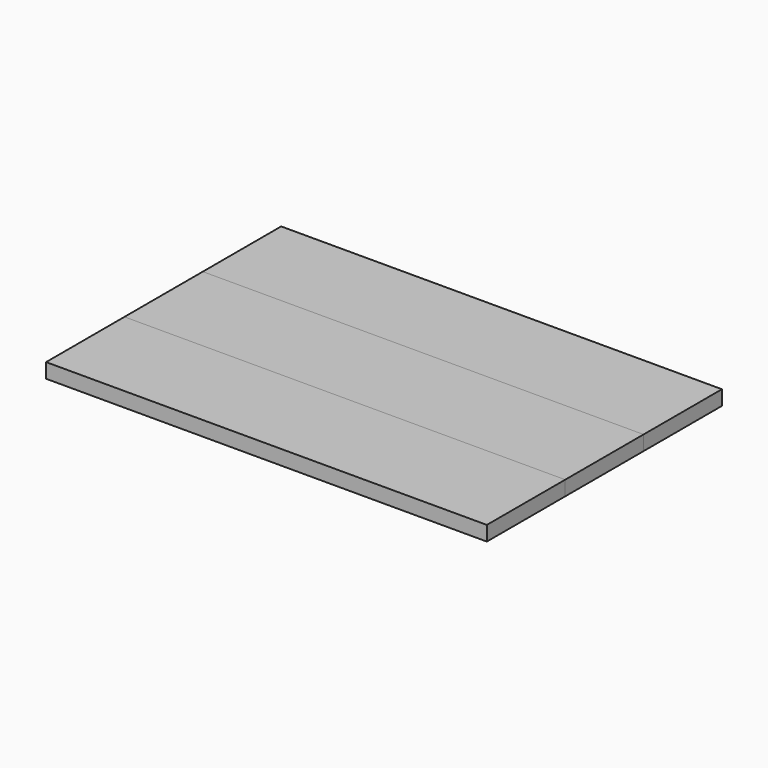
from build123d import *

# Parameters (mm, degrees)
F1_W        = 114.3
F1_H        = 25.4
F3_DEPTH    = 3.81
F4_DEPTH    = 2.54
F5_T1_DEPTH = 13.0403255158


# Not quite as in the source:
# - a fillet or chamfer that OpenCascade refuses, or shapes differently, is made with other operations: its cross-section is extruded or revolved along the edge and cut away or added


with BuildPart() as f3:
    # F1 (on Top) → F3 (new body)
    with BuildSketch(Plane.XY):
        Rectangle(F1_W, F1_H)
    extrude(amount=F3_DEPTH)

    # F2 (on face) → F4 (cut)
    with BuildSketch(Plane.XY):
        Polygon((15.875, 4.7625), (15.875, 3.175), (-15.875, 3.175), (-15.875, 4.7625), (-50.8, 4.7625), (-50.8, -4.7625), (-15.875, -4.7625), (-15.875, -3.175), (15.875, -3.175), (15.875, -4.7625), (50.8, -4.7625), (50.8, 4.7625), align=None)
    extrude(amount=F4_DEPTH, mode=Mode.SUBTRACT)

    # F5: fillet of radius 6.35 on 4 edges, made by hand

    # F5_s2 → F5_t1 (cut)
    with BuildSketch(Plane.XY.offset(-10.5003255158)):
        with BuildLine():
            ThreePointArc((11.6748697937, -3.175), (13.919933824, -3.5851188985), (15.875, -4.7625))
            Line((15.875, -4.7625), (15.875, -3.175))
            Line((15.875, -3.175), (11.6748697937, -3.175))
        make_face()
        with BuildLine():
            ThreePointArc((15.875, 4.7625), (13.919933824, 3.5851188985), (11.6748697937, 3.175))
            Line((11.6748697937, 3.175), (15.875, 3.175))
            Line((15.875, 3.175), (15.875, 4.7625))
        make_face()
        with BuildLine():
            ThreePointArc((-15.875, -4.7625), (-13.919933824, -3.5851188985), (-11.6748697937, -3.175))
            Line((-11.6748697937, -3.175), (-15.875, -3.175))
            Line((-15.875, -3.175), (-15.875, -4.7625))
        make_face()
        with BuildLine():
            ThreePointArc((-11.6748697937, 3.175), (-13.919933824, 3.5851188985), (-15.875, 4.7625))
            Line((-15.875, 4.7625), (-15.875, 3.175))
            Line((-15.875, 3.175), (-11.6748697937, 3.175))
        make_face()
    extrude(amount=F5_T1_DEPTH, mode=Mode.SUBTRACT)


with BuildPart() as f6_1:
    # F6: copy of F3
    add(f3.part.moved(Location((0, 25.4, 0))))


with BuildPart() as f7_1:
    # F7: copy of F3
    add(f3.part.moved(Location((0, -25.4, 0))))


solid = Compound([f3.part, f6_1.part, f7_1.part])
